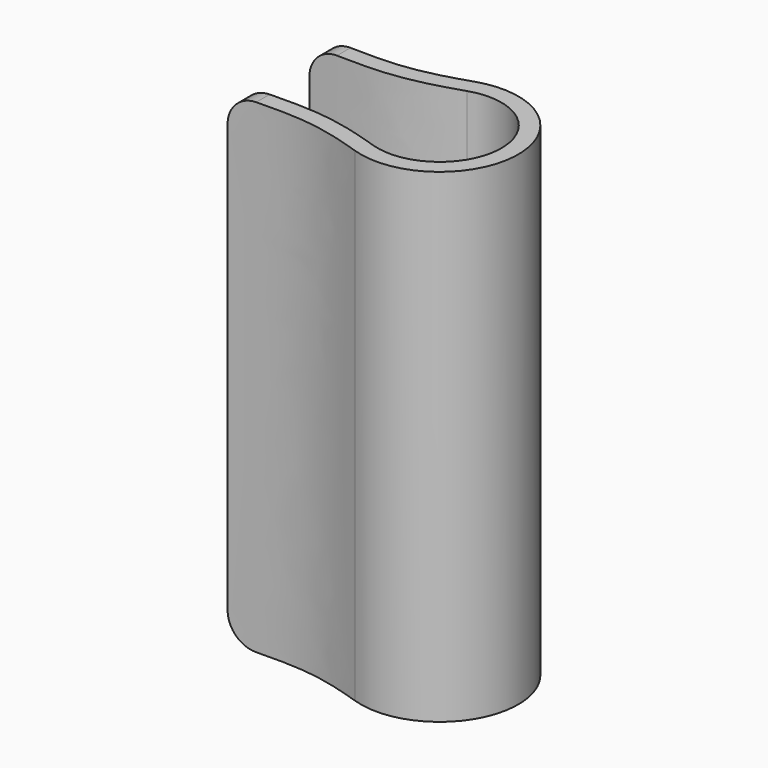
from build123d import *

# Parameters (mm, degrees)
F1_DEPTH = 86.11
F2_R     = 5
F3_R     = 5
F4_R     = 5


# Not quite as in the source:
# - the dataset's text gives a spline's control points without its knots; the knots are read off the source's solid


with BuildPart() as f1:
    # F0 (on Top) → F1 (new body)
    with BuildSketch(Plane.XY):
        with BuildLine():
            add(Edge.make_bspline(
                [(-29.23, -10.585), (-17.4530325989, -10.3312646709), (-14.3938385965, -9.9964864644), (-4.3826738853, -13.2963216573)],
                knots=[0, 0, 0, 0, 24.9948170664, 24.9948170664, 24.9948170664, 24.9948170664], degree=3))
            ThreePointArc((-4.3826738853, -13.2963216573), (14, 0), (-4.3826738853, 13.2963216573))
            add(Edge.make_bspline(
                [(-29.23, 10.585), (-17.4530325989, 10.3312646709), (-14.3938385965, 9.9964864644), (-4.3826738853, 13.2963216573)],
                knots=[0, 0, 0, 0, 24.9948170664, 24.9948170664, 24.9948170664, 24.9948170664], degree=3))
            Line((-29.23, 10.585), (-29.23, 7.5843010349))
            add(Edge.make_bspline(
                [(-29.2300000018, 7.5843009524), (-26.3264289999, 7.5214949579), (-22.7397747479, 7.4189906626), (-18.7158912708, 7.4405712538), (-15.8829489535, 7.5882179461), (-13.0899113875, 7.919906296), (-10.2045998481, 8.4774191522), (-7.0815280556, 9.2907869197), (-4.7236583696, 10.0251594583), (-3.443529459, 10.447109806)],
                knots=[0.0018385431, 0.0018385431, 0.0018385431, 0.0018385431, 0.25, 0.375, 0.5, 0.625, 0.75, 0.875, 1, 1, 1, 1], degree=3))
            ThreePointArc((-3.443529459, 10.447109806), (10.9999999288, 0), (-3.443529459, -10.447109806))
            add(Edge.make_bspline(
                [(-29.2300000018, -7.5843009524), (-26.3264289999, -7.5214949579), (-22.7397747479, -7.4189906626), (-18.7158912708, -7.4405712538), (-15.8829489535, -7.5882179461), (-13.0899113875, -7.919906296), (-10.2045998481, -8.4774191522), (-7.0815280556, -9.2907869197), (-4.7236583696, -10.0251594583), (-3.443529459, -10.447109806)],
                knots=[0.0018385431, 0.0018385431, 0.0018385431, 0.0018385431, 0.25, 0.375, 0.5, 0.625, 0.75, 0.875, 1, 1, 1, 1], degree=3))
            Line((-29.23, -7.5843010349), (-29.23, -10.585))
        make_face()
    extrude(amount=F1_DEPTH)

    # F2
    f2_edges = [f1.edges().sort_by_distance(p)[0] for p in [
        (-29.23, -9.084651, 0),
    ]]
    fillet(f2_edges, radius=F2_R)

    # F3
    f3_edges = [f1.edges().sort_by_distance(p)[0] for p in [
        (-29.23, 9.084651, 0),
    ]]
    fillet(f3_edges, radius=F3_R)

    # F4
    f4_edges = [f1.edges().sort_by_distance(p)[0] for p in [
        (-29.23, -9.084651, 86.11),
        (-29.23, 9.084651, 86.11),
    ]]
    fillet(f4_edges, radius=F4_R)


solid = f1.part
